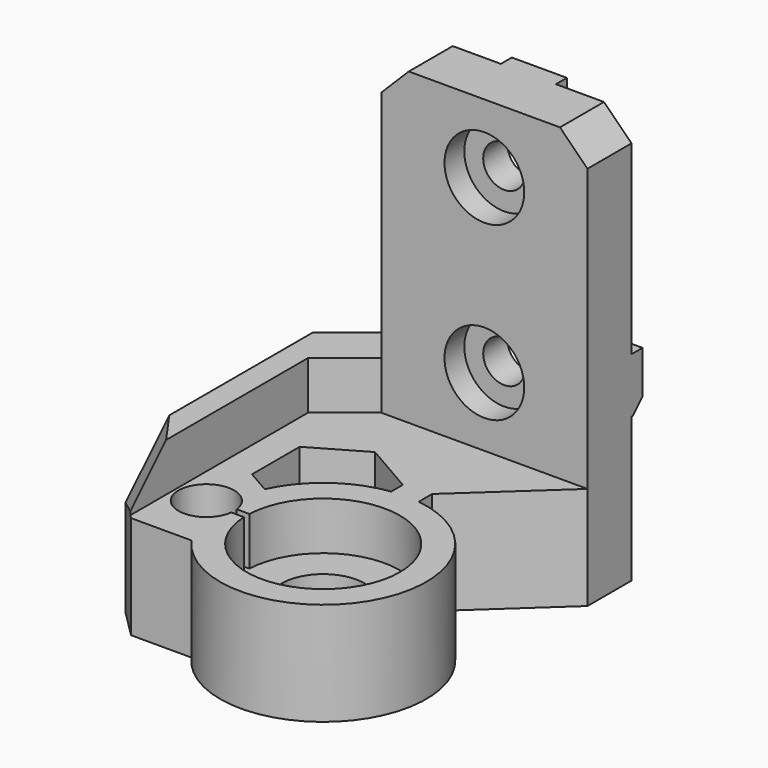
from build123d import *

# Parameters (mm, degrees)
F0_W           = 30
F0_H           = 60
F1_DEPTH       = 8
F2_D           = 6.1
F2_CBORE_D     = 11.6
F2_CBORE_DEPTH = 3.6
F3_R           = 6
F4_DEPTH       = 15
F6_DEPTH       = 12
F5_R           = 6
F7_DEPTH       = 7
F9_DEPTH       = 7
F10_SIZE       = 7
F11_W          = 8
F11_H          = 5
F11_W_2        = 10
F11_H_2        = 8
F12_DEPTH      = 2
F13_SIZE2      = 1.678189
F13_SIZE       = 1.99999
F13_2_SIZE2    = 1.678189
F13_2_SIZE     = 1.99999
F14_SIZE2      = 1.75
F14_SIZE       = 1.75
F15_T1_DEPTH   = 35.5734639037
F16_SIZE       = 3.49999
F17_SIZE       = 4


# Not quite as in the source:
# - a fillet or chamfer that OpenCascade refuses, or shapes differently, is made with other operations: its cross-section is extruded or revolved along the edge and cut away or added
# - a fillet or chamfer is up to 0.001 mm smaller than in the source, because OpenCascade refuses the exact size


with BuildPart() as f1:
    # F0 (on Front) → F1 (new body)
    with BuildSketch(Plane.XZ):
        with Locations((15, 30)):
            Rectangle(F0_W, F0_H)
    extrude(amount=-F1_DEPTH)

    # F2 (through all)
    with Locations(Plane.XZ):
        with Locations((15, 50), (15, 25)):
            CounterBoreHole(F2_D / 2, F2_CBORE_D / 2, F2_CBORE_DEPTH)

    # F3 (on face) → F4 (join)
    with BuildSketch(Plane(origin=(0, 0, 0), x_dir=(1, 0, 0), z_dir=(0, 0, -1))):
        with BuildLine():
            Line((-10, 0), (0, -8))
            Line((0, -8), (0, 0))
            Line((0, 0), (30, 0))
            Line((30, 0), (17, 12))
            Line((17, 12), (17, 14.4339312527))
            ThreePointArc((17, 14.4339312527), (27.843214237, 37.0493127477), (2.7807528874, 38))
            Line((2.7807528874, 38), (-10, 38))
            Line((-10, 38), (-10, 0))
        make_face()
        Polygon((-2, 12.3301270189), (-2, 20.9903810568), (1.4069435951, 22.9573808585), (5.5, 25.3205080757), (13, 20.9903810568), (13, 14.4339312527), (13, 12.3301270189), (5.5, 8), align=None, mode=Mode.SUBTRACT)
        with Locations((15, 29.3)):
            Circle(F3_R, mode=Mode.SUBTRACT)
        with BuildLine():
            Line((5.5, 25.3205080757), (1.4069435951, 22.9573808585))
            ThreePointArc((1.4069435951, 22.9573808585), (6.1147228345, 17.2148086613), (13, 14.4339312527))
            Line((13, 14.4339312527), (13, 20.9903810568))
            Line((13, 20.9903810568), (5.5, 25.3205080757))
        make_face()
    extrude(amount=-F4_DEPTH)

    # F5 (on face) → F6 (cut)
    with BuildSketch(Plane.XY.offset(15)):
        with BuildLine():
            ThreePointArc((2.0190172928, -29.8), (2.0422469022, -29.5504795042), (2.05, -29.3))
            ThreePointArc((2.05, -29.3), (2.0422469022, -29.0495204958), (2.0190172928, -28.8))
            ThreePointArc((2.0190172928, -28.8), (-6.05, -29.3), (2.0190172928, -29.8))
        make_face()
    extrude(amount=-F6_DEPTH, mode=Mode.SUBTRACT)

    # F5 (on face) → F7 (cut)
    with BuildSketch(Plane.XY.offset(15)):
        with BuildLine():
            ThreePointArc((2.0190172928, -28.8), (2.0422469022, -29.0495204958), (2.05, -29.3))
            ThreePointArc((2.05, -29.3), (2.0422469022, -29.5504795042), (2.0190172928, -29.8))
            Line((2.0190172928, -29.8), (3.8612164039, -29.8))
            ThreePointArc((3.8612164039, -29.8), (3.85, -29.3), (3.8612164039, -28.8))
            Line((3.8612164039, -28.8), (2.0190172928, -28.8))
        make_face()
        with BuildLine():
            ThreePointArc((26.15, -29.3), (15.2500628959, -18.1528044537), (3.8612164039, -28.8))
            ThreePointArc((3.8612164039, -28.8), (3.85, -29.3), (3.8612164039, -29.8))
            ThreePointArc((3.8612164039, -29.8), (15.2500628959, -40.4471955463), (26.15, -29.3))
        make_face()
        with Locations((15, -29.3)):
            Circle(F5_R, mode=Mode.SUBTRACT)
        with Locations((15, -29.3)):
            Circle(F5_R)
    extrude(amount=-F7_DEPTH, mode=Mode.SUBTRACT)

    # F8 (on face) → F9 (join)
    with BuildSketch(Plane.XY.offset(15)):
        Polygon((-6.5, -5.2), (0, 0), (0, 8), (-10, 0), (-10, -38), (-6.5, -38), align=None)
    extrude(amount=F9_DEPTH)

    # F10
    f10_edges = [f1.edges().sort_by_distance(p)[0] for p in [
        (-8.25, -38, 22),
    ]]
    chamfer(f10_edges, length=F10_SIZE)

    # F11 (on face) → F12 (join)
    with BuildSketch(Plane(origin=(0, 8, 0), x_dir=(-1, 0, 0), z_dir=(0, 1, 0))):
        with Locations((-15, 57.5)):
            Rectangle(F11_W, F11_H)
        with Locations((-15, 42.5)):
            Rectangle(F11_W, F11_H)
        Polygon((0, 22), (0, 29), (-10, 29), (-10, 21), (0, 21), align=None)
        with Locations((-25, 25)):
            Rectangle(F11_W_2, F11_H_2)
    extrude(amount=F12_DEPTH)

    # F13 (size 2 and 1.6781992624 in the source; OpenCascade refuses exactly that, so slightly less here)
    f13_edges = [f1.edges().sort_by_distance(p)[0] for p in [
        (15, 10, 55),
    ]]
    f13_side = f1.faces().sort_by_distance((15, 9, 55))[0]
    chamfer(f13_edges, length=F13_SIZE, length2=F13_SIZE2, reference=f13_side)

    # F13#2 (size 2 and 1.6781992624 in the source; OpenCascade refuses exactly that, so slightly less here)
    f13_2_edges = [f1.edges().sort_by_distance(p)[0] for p in [
        (15, 10, 40),
    ]]
    f13_2_side = f1.faces().sort_by_distance((15, 9, 40))[0]
    chamfer(f13_2_edges, length=F13_2_SIZE, length2=F13_2_SIZE2, reference=f13_2_side)

    # F14
    f14_edges = [f1.edges().sort_by_distance(p)[0] for p in [
        (25, 10, 21),
        (5, 10, 21),
    ]]
    chamfer(f14_edges, length=F14_SIZE, length2=F14_SIZE2)

    # F15: chamfer of 4 on 1 edges, made by hand

    # F15_s2 → F15_t1 (cut)
    with BuildSketch(Plane.XY.offset(-10.2867319519)):
        Polygon((-6, -38), (-10, -34), (-10, -38), align=None)
    extrude(amount=F15_T1_DEPTH, mode=Mode.SUBTRACT)

    # F16 (size 3.5 in the source; OpenCascade refuses exactly that, so slightly less here)
    f16_edges = [f1.edges().sort_by_distance(p)[0] for p in [
        (-10, -32.5, 20.5),
    ]]
    chamfer(f16_edges, length=F16_SIZE)

    # F17
    f17_edges = [f1.edges().sort_by_distance(p)[0] for p in [
        (30, 4, 60),
        (0, 4, 60),
    ]]
    chamfer(f17_edges, length=F17_SIZE)


solid = f1.part
